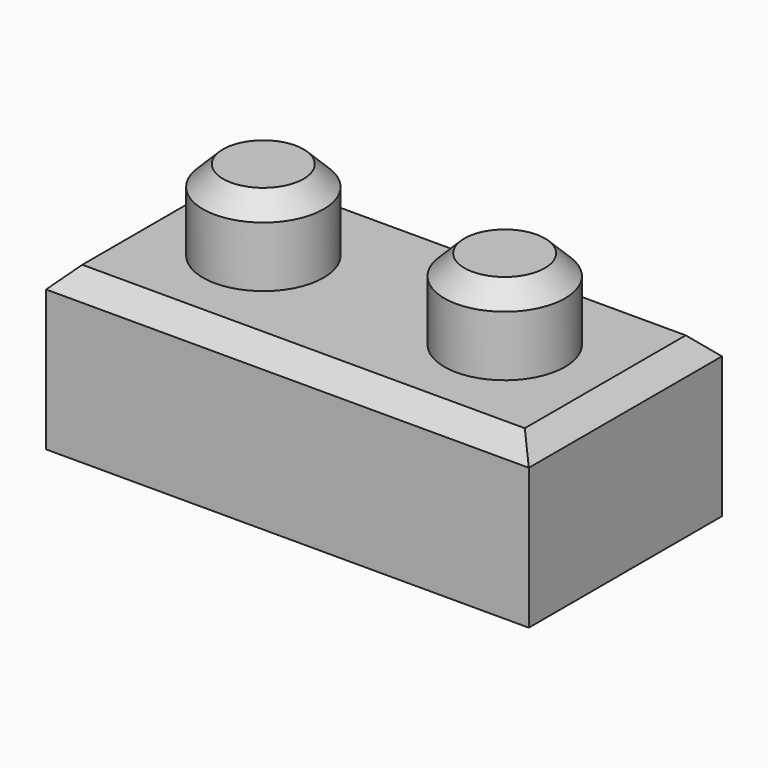
from build123d import *

# Parameters (mm, degrees)
F0_W     = 76.2
F0_H     = 38.1
F1_DEPTH = 25.4
F2_R     = 9.525
F3_DEPTH = 12.7
F4_SIZE2 = 3.175
F4_SIZE  = 3.175
F5_T     = 7.9375


# Not quite as in the source:
# - a shell that OpenCascade refuses in one call is made with other operations: the cavity is built on its own and cut out


with BuildPart() as f1:
    # F0 (on Top) → F1 (new body)
    with BuildSketch(Plane.XY):
        with Locations((38.1, -19.05)):
            Rectangle(F0_W, F0_H)
    extrude(amount=F1_DEPTH)

    # F2 (on face) → F3 (join)
    with BuildSketch(Plane.XY.offset(25.4)):
        with Locations((19.05, -19.05)):
            Circle(F2_R)
        with Locations((57.15, -19.05)):
            Circle(F2_R)
    extrude(amount=F3_DEPTH)

    # F4
    f4_edges = [f1.edges().sort_by_distance(p)[0] for p in [
        (47.625, -19.05, 38.1),
        (9.525, -19.05, 38.1),
        (38.1, -38.1, 25.4),
        (76.2, -19.05, 25.4),
        (38.1, 0, 25.4),
        (0, -19.05, 25.4),
    ]]
    chamfer(f4_edges, length=F4_SIZE, length2=F4_SIZE2)

    # F5: shell of thickness 7.9375, made by hand


with BuildPart() as f5_core1:
    # F5_t2: copy of F1
    add(f1.part)

    # the walls: a layer under each face that stays
    f5_faces = [f5_core1.faces().sort_by_distance(p)[0] for p in [
        (38.1, 0, 11.1125),
        (76.2, -19.05, 11.1125),
        (38.1, -1.5875, 23.8125),
        (0, -19.05, 11.1125),
        (38.1, -38.1, 11.1125),
        (74.6125, -19.05, 23.8125),
        (38.1, -19.05, 25.4),
        (1.5875, -19.05, 23.8125),
        (38.1, -36.5125, 23.8125),
        (9.525, -19.05, 30.1625),
        (47.625, -19.05, 30.1625),
        (11.1125, -19.05, 36.5125),
        (49.2125, -19.05, 36.5125),
        (19.05, -19.05, 38.1),
        (57.15, -19.05, 38.1),
    ]]
    thicken(f5_faces, amount=-F5_T, mode=Mode.SUBTRACT)

    # F5_s3 → F5_t4 (revolve, cut)
    with BuildSketch(Plane.XZ.offset(19.05)):
        Polygon((28.654375, 25.479375), (28.575, 17.4625), (20.6375, 17.4625), (20.6375, 25.4), align=None)
    revolve(axis=Axis((19.05, -19.05, 25.4), (0, 0, 1)), mode=Mode.SUBTRACT)

    # F5_s5 → F5_t6 (revolve, cut)
    with BuildSketch(Plane.XZ.offset(19.05)):
        Polygon((66.754375, 25.479375), (66.675, 17.4625), (58.7375, 17.4625), (58.7375, 25.4), align=None)
    revolve(axis=Axis((57.15, -19.05, 25.4), (0, 0, 1)), mode=Mode.SUBTRACT)


with BuildPart() as f1_1:
    add(f1.part)

    # what is left inside the walls is the cavity
    f5_cavity = [f5_core1.part.solids().sort_by_distance(p)[0] for p in [
        (38.1, -22.754167, 0.079375),
    ]]
    add(f5_cavity, mode=Mode.SUBTRACT)


solid = f1_1.part
